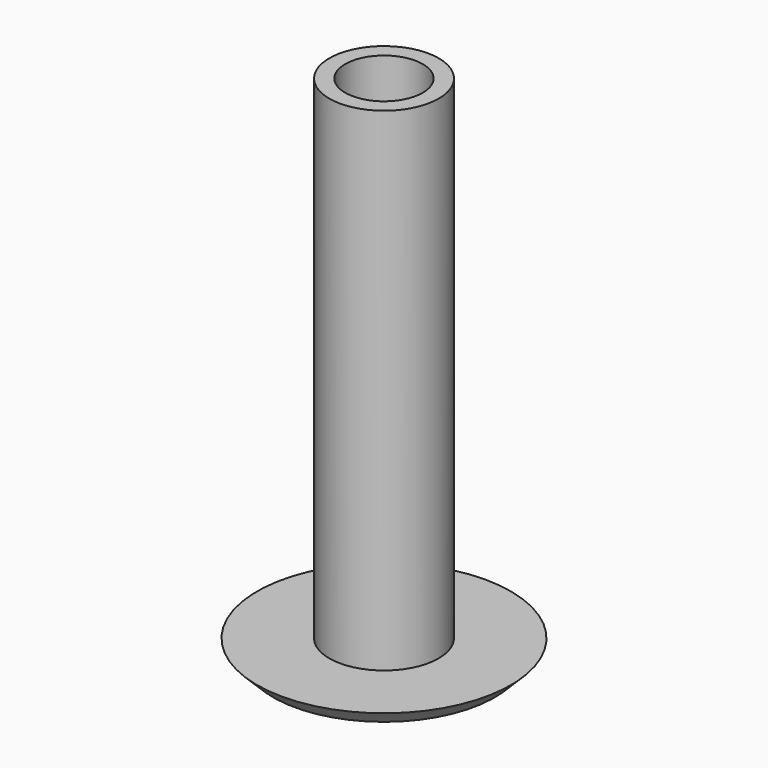
from build123d import *

# Parameters (mm, degrees)
F3_DEPTH = 5
F1_R     = 17.2
F4_DEPTH = 160
F0_R     = 12.2
F5_DEPTH = 160


# Not quite as in the source:
# - a fillet or chamfer that OpenCascade refuses, or shapes differently, is made with other operations: its cross-section is extruded or revolved along the edge and cut away or added


with BuildPart() as f3:
    # F2 (on Top) → F3 (new body)
    with BuildSketch(Plane.XY):
        with BuildLine():
            ThreePointArc((40, 0), (28.2842712475, 28.2842712475), (0, 40))
            ThreePointArc((0, 40), (-28.2842712475, 28.2842712475), (-40, 0))
            ThreePointArc((-40, 0), (-28.2842712475, -28.2842712475), (0, -40))
            ThreePointArc((0, -40), (28.2842712475, -28.2842712475), (40, 0))
        make_face()
    extrude(amount=F3_DEPTH)

    # F1 (on Top) → F4 (join)
    with BuildSketch(Plane.XY):
        Circle(F1_R)
    extrude(amount=F4_DEPTH)

    # F0 (on Top) → F5 (cut)
    with BuildSketch(Plane.XY):
        Circle(F0_R)
    extrude(amount=F5_DEPTH, mode=Mode.SUBTRACT)

    # F6: chamfer of 5.08 on 1 edges, made by hand

    # F6_s1 → F6_t2 (revolve, cut)
    with BuildSketch(Plane.YZ):
        Polygon((40, 5.08), (34.92, 0), (40, 0), align=None)
    revolve(axis=Axis((0, 0, 0), (0, 0, 1)), mode=Mode.SUBTRACT)


solid = f3.part
